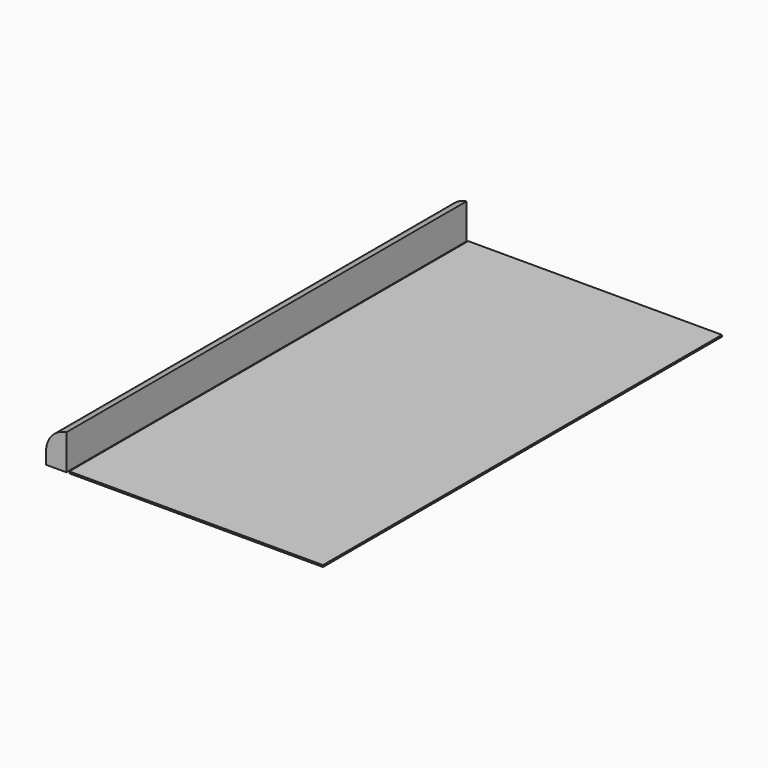
from build123d import *

# Parameters (mm, degrees)
F1_W        = 5.8504454792
F1_H        = 144.171692431
F2_DEPTH    = 10.16
F0_W        = 73.1305684894
F0_H        = 143.7538042665
F3_DEPTH    = 0.508
F4_T1_DEPTH = 177.600144384


# Not quite as in the source:
# - a fillet or chamfer that OpenCascade refuses, or shapes differently, is made with other operations: its cross-section is extruded or revolved along the edge and cut away or added


with BuildPart() as f2:
    # F1 (on Top) → F2 (new body)
    with BuildSketch(Plane.XY):
        with Locations((-57.8831378371, 2.1721757948)):
            Rectangle(F1_W, F1_H)
    extrude(amount=F2_DEPTH)

    # F4: fillet of radius 6.7453126933 on 1 edges, made by hand

    # F4_s2 → F4_t1 (cut)
    with BuildSketch(Plane.XZ.offset(-90.9722479869)):
        with BuildLine():
            ThreePointArc((-60.8083605766, 3.4743096094), (-59.1392375227, 7.9163296539), (-54.9579150975, 10.16))
            Line((-54.9579150975, 10.16), (-60.8083605766, 10.16))
            Line((-60.8083605766, 10.16), (-60.8083605766, 3.4743096094))
        make_face()
    extrude(amount=F4_T1_DEPTH, mode=Mode.SUBTRACT)


with BuildPart() as f3:
    # F0 (on Top) → F3 (new body)
    with BuildSketch(Plane.XY):
        with Locations((-17.5568545237, 1.9632317126)):
            Rectangle(F0_W, F0_H)
    extrude(amount=F3_DEPTH)


solid = Compound([f2.part, f3.part])
